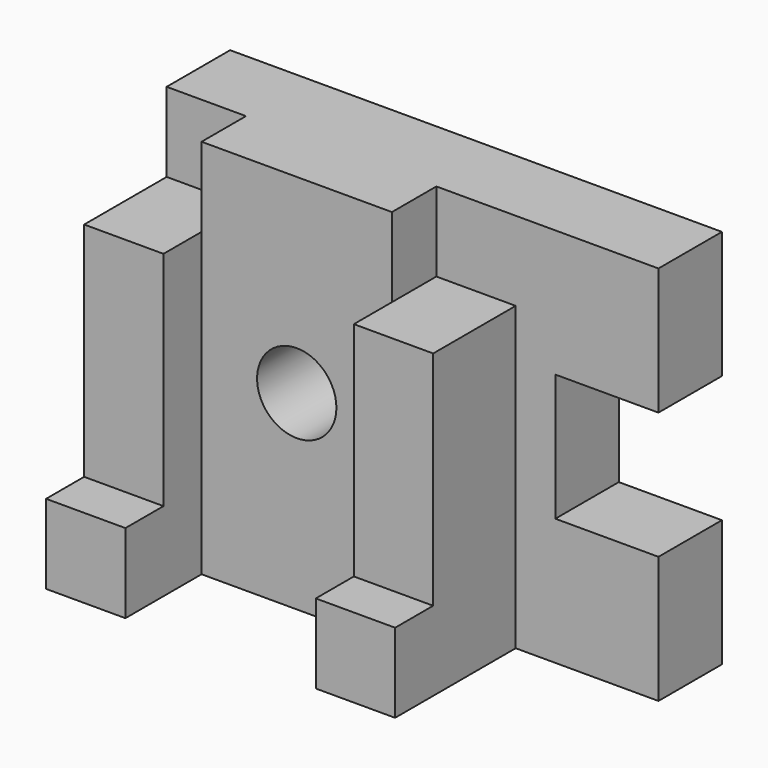
from build123d import *

# Parameters (mm, degrees)
F0_W     = 31.75
F0_H     = 88.9
F0_H_2   = 31.75
F0_R     = 15.875
F1_DEPTH = 31.75
F2_DEPTH = 73.025
F3_DEPTH = 73.025
F4_DEPTH = 92.075
F5_DEPTH = 53.975


# Not quite as in the source:
# - a feature names something its author has since deleted; it is built from what else it names


with BuildPart() as f1:
    # F0 (on Front) → F1 (new body)
    with BuildSketch(Plane.XZ):
        Polygon((114.6503422856, 101.6), (57.5003422856, 101.6), (57.5003422856, 69.85), (57.5003422856, -19.05), (57.5003422856, -50.8), (114.6503422856, -50.8), (114.6503422856, 0), (73.3753422856, 0), (73.3753422856, 50.8), (114.6503422856, 50.8), align=None)
        with Locations((41.6253422856, 25.4)):
            Rectangle(F0_W, F0_H)
        with Locations((41.6253422856, -34.925)):
            Rectangle(F0_W, F0_H_2)
        Polygon((-12.3496577144, 101.6), (-50.4496577144, 101.6), (-50.4496577144, 69.85), (-50.4496577144, -19.05), (-50.4496577144, -50.8), (25.7503422856, -50.8), (25.7503422856, -19.05), (25.7503422856, 69.85), (25.7503422856, 101.6), align=None)
        with Locations((-12.3496577144, 25.4)):
            Circle(F0_R, mode=Mode.SUBTRACT)
        with Locations((-66.3246577144, 25.4)):
            Rectangle(F0_W, F0_H)
        with Locations((-66.3246577144, -34.925)):
            Rectangle(F0_W, F0_H_2)
        with Locations((-66.3246577144, 85.725)):
            Rectangle(F0_W, F0_H_2)
        with Locations((41.6253422856, 85.725)):
            Rectangle(F0_W, F0_H_2)
    extrude(amount=F1_DEPTH)

    # F0 (on Front) → F2 (join)
    with BuildSketch(Plane.XZ):
        with Locations((-66.3246577144, 25.4)):
            Rectangle(F0_W, F0_H)
        with Locations((-66.3246577144, -34.925)):
            Rectangle(F0_W, F0_H_2)
    extrude(amount=F2_DEPTH)

    # F0 (on Front) → F3 (join)
    with BuildSketch(Plane.XZ):
        with Locations((41.6253422856, -34.925)):
            Rectangle(F0_W, F0_H_2)
        with Locations((41.6253422856, 25.4)):
            Rectangle(F0_W, F0_H)
    extrude(amount=F3_DEPTH)

    # F0 (on Front) → F4 (join)
    with BuildSketch(Plane.XZ):
        with Locations((-66.3246577144, -34.925)):
            Rectangle(F0_W, F0_H_2)
        with Locations((41.6253422856, -34.925)):
            Rectangle(F0_W, F0_H_2)
    extrude(amount=F4_DEPTH)

    # F0 (on Front) → F5 (join)
    with BuildSketch(Plane.XZ):
        Polygon((-12.3496577144, 101.6), (-50.4496577144, 101.6), (-50.4496577144, 69.85), (-50.4496577144, -19.05), (-50.4496577144, -50.8), (25.7503422856, -50.8), (25.7503422856, -19.05), (25.7503422856, 69.85), (25.7503422856, 101.6), align=None)
        with Locations((-12.3496577144, 25.4)):
            Circle(F0_R, mode=Mode.SUBTRACT)
    extrude(amount=F5_DEPTH)


solid = f1.part
